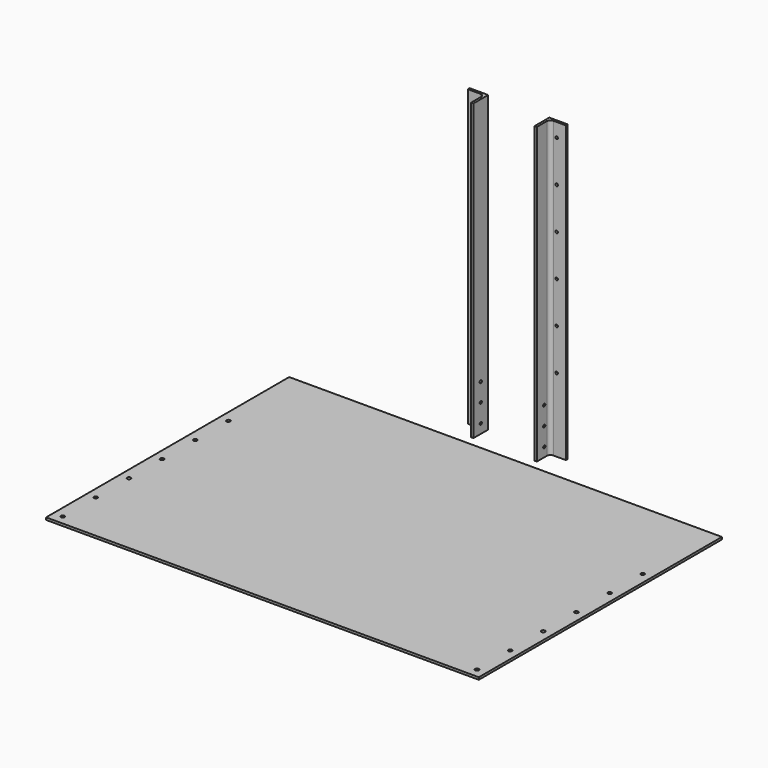
from build123d import *

# Parameters (mm, degrees)
F1_DEPTH = 406.4
F2_R     = 5.08
F3_R     = 1.905
F4_DEPTH = 25.401
F5_R     = 1.778
F6_DEPTH = 25.401
F8_W     = 596.9
F8_H     = 419.1
F8_R     = 2.5527
F9_DEPTH = 3.175


# Not quite as in the source:
# - a length typed as a fraction of an inch, garbled in the dataset ("3 / 203.2 mm" for 3/8 in), is restored


with BuildPart() as f1:
    # F0 (on Top) → F1 (new body)
    with BuildSketch(Plane.XY):
        Polygon((42.1772189438, 44.9829958379), (42.1772189438, 19.5829958379), (45.3522189438, 19.5829958379), (45.3522189438, 41.8079958379), (67.5772189438, 41.8079958379), (67.5772189438, 44.9829958379), align=None)
    extrude(amount=F1_DEPTH)

    # F2
    f2_edges = [f1.edges().sort_by_distance(p)[0] for p in [
        (45.352219, 41.807996, 203.2),
    ]]
    fillet(f2_edges, radius=F2_R)

    # F3 (on face) → F4 (cut, through all)
    with BuildSketch(Plane(origin=(42.1772189438, 0, 0), x_dir=(0, -1, 0), z_dir=(-1, 0, 0))):
        with Locations((-32.2829958379, 12.7)):
            Circle(F3_R)
        with Locations((-32.2829958379, 38.1)):
            Circle(F3_R)
        with Locations((-32.2829958379, 63.5)):
            Circle(F3_R)
    extrude(amount=-F4_DEPTH, mode=Mode.SUBTRACT)

    # F5 (on face) → F6 (cut, through all)
    with BuildSketch(Plane(origin=(0, 44.9829958379, 0), x_dir=(-1, 0, 0), z_dir=(0, 1, 0))):
        with Locations((-54.8772189438, 101.6)):
            Circle(F5_R)
        with Locations((-54.8772189438, 158.75)):
            Circle(F5_R)
        with Locations((-54.8772189438, 215.9)):
            Circle(F5_R)
        with Locations((-54.8772189438, 273.05)):
            Circle(F5_R)
        with Locations((-54.8772189438, 330.2)):
            Circle(F5_R)
        with Locations((-54.8772189438, 387.35)):
            Circle(F5_R)
    extrude(amount=-F6_DEPTH, mode=Mode.SUBTRACT)


with BuildPart() as f7_1:
    # F7: instance of F1
    add(f1.part.mirror(Plane.YZ))


with BuildPart() as f9:
    # F8 (on Top) → F9 (new body)
    with BuildSketch(Plane.XY):
        with Locations((16.0670019686, -207.3692955732)):
            Rectangle(F8_W, F8_H)
        with Locations((-269.6829980314, -404.2192955732)):
            Circle(F8_R, mode=Mode.SUBTRACT)
        with Locations((-269.6829980314, -347.0692955732)):
            Circle(F8_R, mode=Mode.SUBTRACT)
        with Locations((-269.6829980314, -289.9192955732)):
            Circle(F8_R, mode=Mode.SUBTRACT)
        with Locations((-269.6829980314, -232.7692955732)):
            Circle(F8_R, mode=Mode.SUBTRACT)
        with Locations((301.8170019686, -404.2192955732)):
            Circle(F8_R, mode=Mode.SUBTRACT)
        with Locations((301.8170019686, -347.0692955732)):
            Circle(F8_R, mode=Mode.SUBTRACT)
        with Locations((301.8170019686, -289.9192955732)):
            Circle(F8_R, mode=Mode.SUBTRACT)
        with Locations((301.8170019686, -232.7692955732)):
            Circle(F8_R, mode=Mode.SUBTRACT)
        with Locations((-269.6829980314, -175.6192955732)):
            Circle(F8_R, mode=Mode.SUBTRACT)
        with Locations((-269.6829980314, -118.4692955732)):
            Circle(F8_R, mode=Mode.SUBTRACT)
        with Locations((301.8170019686, -175.6192955732)):
            Circle(F8_R, mode=Mode.SUBTRACT)
        with Locations((301.8170019686, -118.4692955732)):
            Circle(F8_R, mode=Mode.SUBTRACT)
    extrude(amount=F9_DEPTH)


solid = Compound([f1.part, f7_1.part, f9.part])
